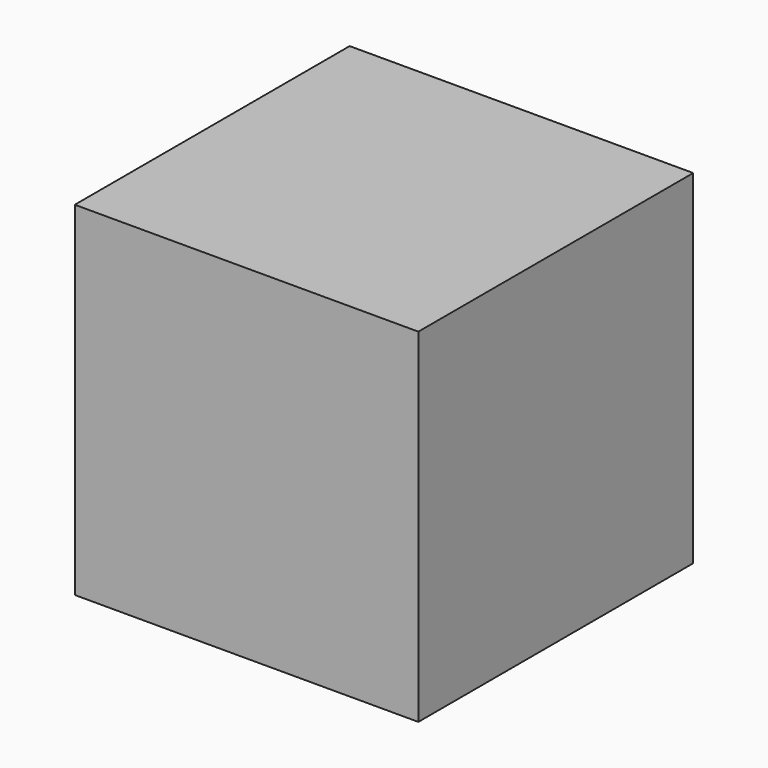
from build123d import *

# Parameters (mm, degrees)
F0_W     = 20
F0_H     = 20
F1_DEPTH = 20
F2_DEPTH = 10
F3_SIZE  = 9.99999
F4_DEPTH = 10
F5_R     = 9.99999


# Not quite as in the source:
# - a fillet or chamfer is up to 0.001 mm smaller than in the source, because OpenCascade refuses the exact size


with BuildPart() as f1:
    # F0 (on Top) → F1 (new body)
    with BuildSketch(Plane.XY):
        with Locations((-0.0724839047, 2.2167936491)):
            Rectangle(F0_W, F0_H)
    extrude(amount=F1_DEPTH)


with BuildPart() as f2:
    # F0 (on Top) → F2 (new body)
    with BuildSketch(Plane.XY):
        with Locations((-0.0724839047, 2.2167936491)):
            Rectangle(F0_W, F0_H)
    extrude(amount=F2_DEPTH)

    # F3 (size 10 in the source; OpenCascade refuses exactly that, so slightly less here)
    f3_edges = [f2.edges().sort_by_distance(p)[0] for p in [
        (-0.072484, 12.216794, 10),
        (-10.072484, 2.216794, 10),
        (-0.072484, -7.783206, 10),
        (9.927516, 2.216794, 10),
    ]]
    chamfer(f3_edges, length=F3_SIZE)


with BuildPart() as f4:
    # F0 (on Top) → F4 (new body)
    with BuildSketch(Plane.XY):
        with Locations((-0.0724839047, 2.2167936491)):
            Rectangle(F0_W, F0_H)
    extrude(amount=F4_DEPTH)

    # F5 (radius 10 in the source; OpenCascade refuses exactly that, so slightly less here)
    f5_edges = [f4.edges().sort_by_distance(p)[0] for p in [
        (-0.072484, 12.216794, 10),
        (-10.072484, 2.216794, 10),
        (-0.072484, -7.783206, 10),
        (9.927516, 2.216794, 10),
    ]]
    fillet(f5_edges, radius=F5_R)


solid = Compound([f1.part, f2.part, f4.part])
